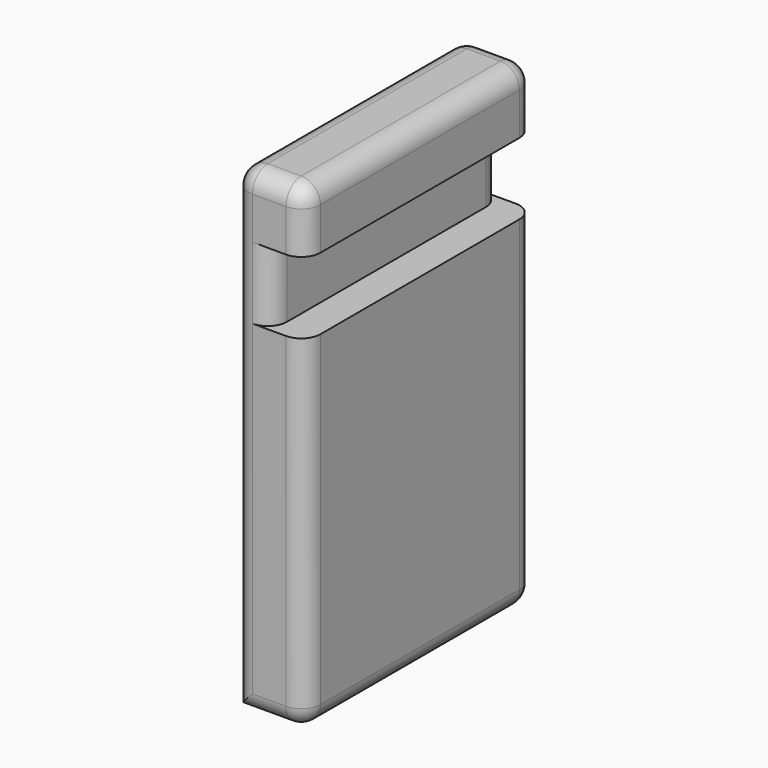
from build123d import *

# Parameters (mm, degrees)
F0_W     = 19.05
F0_H     = 127
F1_DEPTH = 76.2
F2_W     = 76.2
F2_H     = 19.05
F3_DEPTH = 8.89
F4_R     = 5.07999


# Not quite as in the source:
# - a fillet or chamfer is up to 0.001 mm smaller than in the source, because OpenCascade refuses the exact size


with BuildPart() as f1:
    # F0 (on Front) → F1 (new body)
    with BuildSketch(Plane.XZ):
        with Locations((-61.3191734314, 10.0326964855)):
            Rectangle(F0_W, F0_H)
    extrude(amount=F1_DEPTH)

    # F2 (on face) → F3 (cut)
    with BuildSketch(Plane.YZ.offset(-51.7941734314)):
        with Locations((-38.1, 47.7159310818)):
            Rectangle(F2_W, F2_H)
    extrude(amount=-F3_DEPTH, mode=Mode.SUBTRACT)

    # F4 (radius 5.08 in the source; OpenCascade refuses exactly that, so slightly less here)
    f4_edges = [f1.edges().sort_by_distance(p)[0] for p in [
        (-70.844173, -76.2, 10.032696),
        (-51.794173, -76.2, 65.386814),
        (-61.319173, -76.2, 73.532696),
        (-60.684173, -76.2, 47.715931),
        (-60.684173, 0, 47.715931),
        (-51.794173, -76.2, -7.638186),
        (-51.794173, -38.1, -53.467304),
        (-61.319173, -76.2, -53.467304),
        (-61.319173, 0, -53.467304),
        (-51.794173, 0, -7.638186),
        (-70.844173, 0, 10.032696),
        (-51.794173, 0, 65.386814),
        (-61.319173, 0, 73.532696),
        (-51.794173, -38.1, 73.532696),
        (-70.844173, -38.1, 73.532696),
    ]]
    fillet(f4_edges, radius=F4_R)


solid = f1.part
